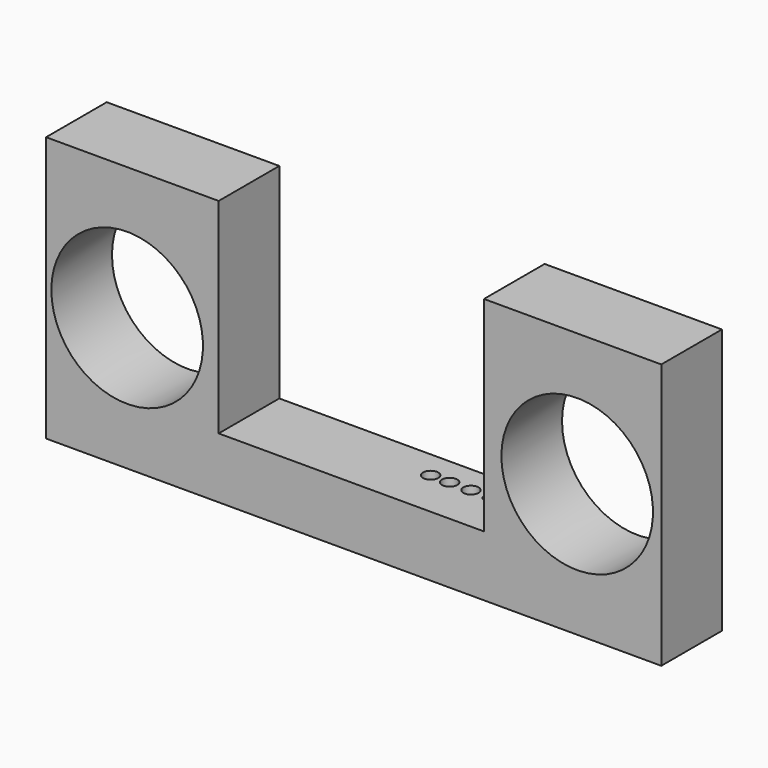
from build123d import *

# Parameters (mm, degrees)
F0_W        = 206.1404287815
F0_H        = 88.9
F1_DEPTH    = 25.4
F4_D        = 50.8
F4_ON_F3_D  = 50.8
F5_W        = 88.9
F5_H        = 68.58
F6_DEPTH    = 25.401
F7_T        = 6.35
F7_T3_DEPTH = 38.1
F9_D        = 5.08
F9_DEPTH    = 3.175
F9_TIP      = 1.5261859723


# Not quite as in the source:
# - a shell that OpenCascade refuses in one call is made with other operations: the cavity is built on its own and cut out


with BuildPart() as f1:
    # F0 (on Front) → F1 (new body)
    with BuildSketch(Plane.XZ):
        Rectangle(F0_W, F0_H)
    extrude(amount=F1_DEPTH)

    # F4 (through all)
    with Locations(Plane.XZ.offset(25.4)):
        with Locations((-75.905919075, 0)):
            Hole(F4_D / 2)

    # F4 on F3 (through all)
    with Locations(Plane.XZ.offset(25.4)):
        with Locations((74.8937055469, 0)):
            Hole(F4_ON_F3_D / 2)

    # F5 (on face) → F6 (cut, through all)
    with BuildSketch(Plane.XZ.offset(25.4)):
        with Locations((-0.7901638031, 10.16)):
            Rectangle(F5_W, F5_H)
    extrude(amount=-F6_DEPTH, mode=Mode.SUBTRACT)

    # F7: shell of thickness 6.35, made by hand


with BuildPart() as f7_core1:
    # F7_t2: copy of F1
    add(f1.part)

    # the walls: a layer under each face that stays
    f7_faces = [f7_core1.faces().sort_by_distance(p)[0] for p in [
        (0, -12.7, -44.45),
        (-103.0702143908, -12.7, 0),
        (103.0702143908, -12.7, 0),
        (-68.7134762605, -25.4, -29.6333333333),
        (-74.1551890969, -12.7, 44.45),
        (73.3650252938, -12.7, 44.45),
        (-45.2401638031, -12.7, 10.16),
        (-0.7901638031, -12.7, -24.13),
        (43.6598361969, -12.7, 10.16),
        (-101.305919075, -12.7, 0),
        (49.4937055469, -12.7, 0),
    ]]
    thicken(f7_faces, amount=-F7_T, mode=Mode.SUBTRACT)

    # F7_s4 → F7_t3 (cut)
    with BuildSketch(Plane.XZ.offset(-6.35)):
        Polygon((-45.1766638031, -24.0665), (-51.5901638031, -24.13), (-51.5901638031, -30.48), (-45.2401638031, -30.48), align=None)
        Polygon((43.5963361969, -24.0665), (43.6598361969, -30.48), (50.0098361969, -30.48), (50.0098361969, -24.13), align=None)
    extrude(amount=F7_T3_DEPTH, mode=Mode.SUBTRACT)


with BuildPart() as f1_1:
    add(f1.part)

    # what is left inside the walls is the cavity
    f7_cavity = [f7_core1.part.solids().sort_by_distance(p)[0] for p in [
        (0, -12.7, -38.0365),
        (-73.404336, -6.35, 31.714994),
        (72.62573, -6.35, 31.732555),
    ]]
    add(f7_cavity, mode=Mode.SUBTRACT)

    # F9
    with Locations(Plane.XY.offset(-24.13)):
        with Locations((40.6420230865, -9.2453807592), (33.507373184, -9.2453807592), (26.3727232814, -9.2453807592), (19.2380733788, -9.2453807592), (12.8678502515, -9.2453807592)):
            Hole(F9_D / 2, depth=F9_DEPTH)
            with Locations((0, 0, -(F9_DEPTH + F9_TIP / 2))):  # 118° drill point
                Cone(0, F9_D / 2, F9_TIP, mode=Mode.SUBTRACT)


solid = f1_1.part
